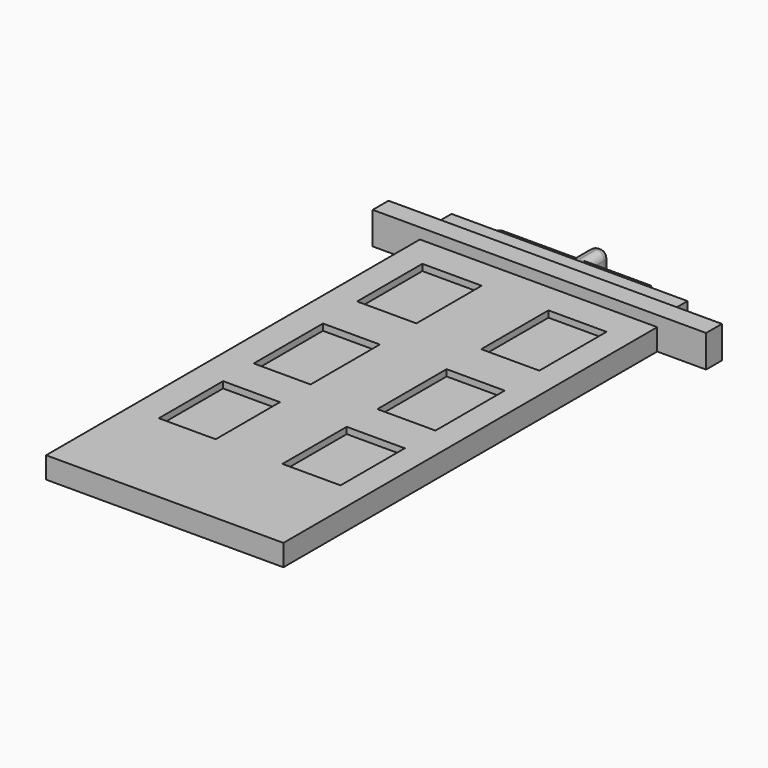
from build123d import *

# Parameters (mm, degrees)
F0_W        = 0.9483136237
F0_H        = 3.3681727946
F0_W_2      = 28.0582979321
F0_H_2      = 55.2397826687
F0_W_3      = 6.7223012447
F0_H_3      = 9.4989053905
F0_H_4      = 10.2295875549
F0_W_4      = 6.8684406579
F0_W_5      = 7.014580071
F0_H_5      = 9.6450410783
F0_H_6      = 9.9373161793
F0_W_6      = 10.7689313591
F0_H_7      = 1.450072974
F0_W_7      = 10.0600272417
F1_DEPTH    = 2.54
F2_R        = 0.889
F3_DEPTH    = 1.778
F4_T4_DEPTH = 15.6041495789
F4_T9_DEPTH = 15.6041495789
F5_DEPTH    = 3.81
F6_DEPTH    = 3.302


# Not quite as in the source:
# - a fillet or chamfer that OpenCascade refuses, or shapes differently, is made with other operations: its cross-section is extruded or revolved along the edge and cut away or added


with BuildPart() as f1:
    # F0 (on Top) → F1 (new body)
    with BuildSketch(Plane.XY):
        with Locations((-55.3537514061, 60.8582701534)):
            Rectangle(F0_W, F0_H)
        Polygon((-69.7804093361, 57.7241107821), (-69.7804093361, 55.3859174252), (-41.8754070997, 55.3859174252), (-41.8754070997, 57.7241107821), (-44.8195673525, 57.7241107821), (-54.8795945942, 57.7241107821), (-55.8279082179, 57.7241107821), (-56.7762218416, 57.7241107821), (-67.5451532006, 57.7241107821), align=None)
        Polygon((-75.3612667322, 53.0477277935), (-69.7804093361, 53.0477277935), (-41.7221114039, 53.0477277935), (-35.9445475042, 53.0477277935), (-35.9445475042, 55.3859174252), (-41.8754070997, 55.3859174252), (-69.7804093361, 55.3859174252), (-75.3612667322, 55.3859174252), align=None)
        with Locations((-56.3020650297, 60.8582701534)):
            Rectangle(F0_W, F0_H)
        with Locations((-55.75126037, 25.4278364591)):
            Rectangle(F0_W_2, F0_H_2)
        with Locations((-62.9119724035, 14.8329045624)):
            Rectangle(F0_W_3, F0_H_3, mode=Mode.SUBTRACT)
        with Locations((-62.9119724035, 29.2273983359)):
            Rectangle(F0_W_3, F0_H_4, mode=Mode.SUBTRACT)
        with Locations((-48.2252072543, 14.8329045624)):
            Rectangle(F0_W_4, F0_H_3, mode=Mode.SUBTRACT)
        with Locations((-48.2252072543, 29.2273983359)):
            Rectangle(F0_W_4, F0_H_4, mode=Mode.SUBTRACT)
        with Locations((-63.0581118166, 44.571781531)):
            Rectangle(F0_W_5, F0_H_5, mode=Mode.SUBTRACT)
        with Locations((-48.2252072543, 44.4256439805)):
            Rectangle(F0_W_4, F0_H_6, mode=Mode.SUBTRACT)
        with Locations((-62.1606875211, 58.4491472691)):
            Rectangle(F0_W_6, F0_H_7)
        with Locations((-55.3537514061, 58.4491472691)):
            Rectangle(F0_W, F0_H_7)
        with Locations((-49.8495809734, 58.4491472691)):
            Rectangle(F0_W_7, F0_H_7)
        with Locations((-56.3020650297, 58.4491472691)):
            Rectangle(F0_W, F0_H_7)
    extrude(amount=F1_DEPTH)

    # F2
    f2_edges = [f1.edges().sort_by_distance(p)[0] for p in [
        (-54.879595, 60.85827, 2.54),
        (-56.776222, 60.85827, 2.54),
        (-55.827908, 62.542357, 2.54),
        (-56.776222, 62.542357, 1.27),
        (-54.879595, 62.542357, 1.27),
    ]]
    fillet(f2_edges, radius=F2_R)

    # F0 (on Top) → F3 (join)
    with BuildSketch(Plane.XY):
        with Locations((-63.0581118166, 44.571781531)):
            Rectangle(F0_W_5, F0_H_5)
        with Locations((-48.2252072543, 44.4256439805)):
            Rectangle(F0_W_4, F0_H_6)
        with Locations((-62.9119724035, 29.2273983359)):
            Rectangle(F0_W_3, F0_H_4)
        with Locations((-48.2252072543, 29.2273983359)):
            Rectangle(F0_W_4, F0_H_4)
        with Locations((-48.2252072543, 14.8329045624)):
            Rectangle(F0_W_4, F0_H_3)
        with Locations((-62.9119724035, 14.8329045624)):
            Rectangle(F0_W_3, F0_H_3)
    extrude(amount=F3_DEPTH)

    # F4: chamfer of 2.54 on 2 edges, made by hand


with BuildPart() as f4_tool2:
    # F4_s3 → F4_t4 (new body)
    with BuildSketch(Plane.XY.offset(-6.5320747894)):
        Polygon((-67.5451532006, 56.6341837561), (-65.0051532006, 59.1741837561), (-67.5451532006, 59.1741837561), align=None)
    extrude(amount=F4_T4_DEPTH)

    split(bisect_by=Plane.XZ.offset(-57.7241107821), keep=Keep.BOTTOM)


with BuildPart() as f1_1:
    add(f1.part)

    # F4_t1: cut F4_tool2
    add(f4_tool2.part, mode=Mode.SUBTRACT)


with BuildPart() as f4_tool7:
    # F4_s8 → F4_t9 (new body)
    with BuildSketch(Plane.XY.offset(-6.5320747894)):
        Polygon((-44.8195673525, 56.6341837561), (-47.3595673525, 59.1741837561), (-44.8195673525, 59.1741837561), align=None)
    extrude(amount=F4_T9_DEPTH)

    split(bisect_by=Plane.XZ.offset(-57.7241107821), keep=Keep.BOTTOM)


with BuildPart() as f1_2:
    add(f1_1.part)

    # F4_t6: cut F4_tool7
    add(f4_tool7.part, mode=Mode.SUBTRACT)

    # F0 (on Top) → F5 (join)
    with BuildSketch(Plane.XY):
        Polygon((-75.3612667322, 53.0477277935), (-69.7804093361, 53.0477277935), (-41.7221114039, 53.0477277935), (-35.9445475042, 53.0477277935), (-35.9445475042, 55.3859174252), (-41.8754070997, 55.3859174252), (-69.7804093361, 55.3859174252), (-75.3612667322, 55.3859174252), align=None)
    extrude(amount=F5_DEPTH)

    # F0 (on Top) → F6 (join)
    with BuildSketch(Plane.XY):
        Polygon((-69.7804093361, 57.7241107821), (-69.7804093361, 55.3859174252), (-41.8754070997, 55.3859174252), (-41.8754070997, 57.7241107821), (-44.8195673525, 57.7241107821), (-54.8795945942, 57.7241107821), (-55.8279082179, 57.7241107821), (-56.7762218416, 57.7241107821), (-67.5451532006, 57.7241107821), align=None)
    extrude(amount=F6_DEPTH)


solid = f1_2.part
